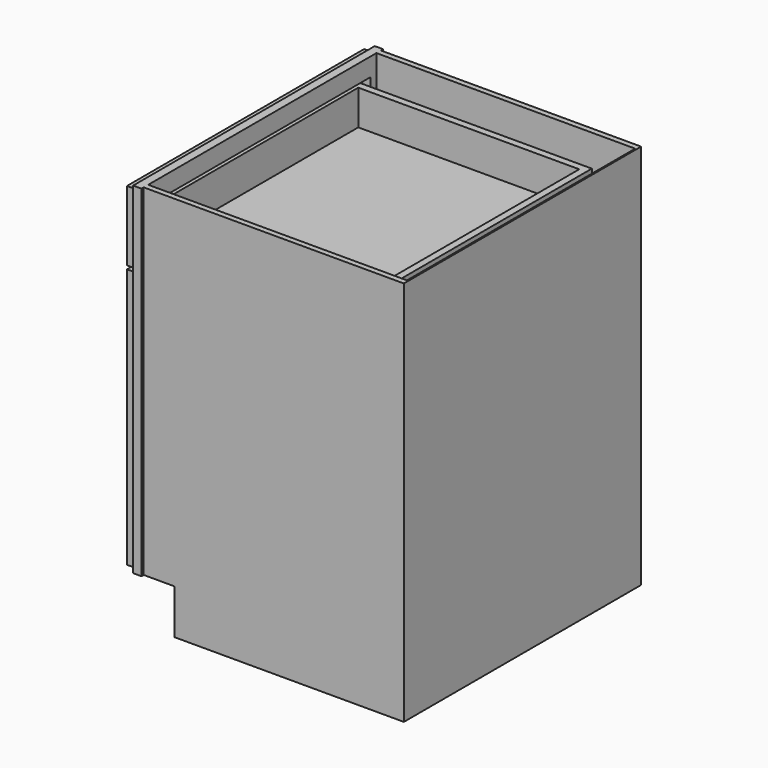
from build123d import *

# Parameters (mm, degrees)
F0_W          = 609.6
F0_H          = 876.3
F1_DEPTH      = 685.8
F2_W          = 88.9
F2_H          = 101.6
F3_DEPTH      = 685.801
F4_W          = 612.7229508197
F4_H          = 692.15
F5_DEPTH      = 19.05
F6_W          = 590.55
F6_H          = 6.35
F7_DEPTH      = 876.301
F8_W          = 587.375
F8_H          = 647.7
F9_DEPTH      = 733.425
F10_W         = 612.7229508197
F10_H         = 41.275
F11_DEPTH     = 19.05
F12_W         = 336.55
F12_H         = 590.5627
F12_W_2       = 222.25
F12_H_2       = 476.2627
F13_DEPTH     = 19.05
F14_W         = 6.35
F14_H         = 222.25
F15_DEPTH     = 476.2627
F16_SIZE      = 3.175
F17_W         = 673.1
F17_H         = 158.75
F17_W_2       = 558.8
F17_H_2       = 82.55
F18_DEPTH     = 19.05
F19_W         = 6.35
F19_H         = 558.8
F20_DEPTH     = 82.55
F21_SIZE      = 3.175
F22_W         = 504.825
F22_H         = 647.7
F23_DEPTH     = 101.6
F24_W         = 584.2
F24_H         = 95.25
F25_DEPTH     = 533.4
F26_T         = 15.875
F26_T3_DEPTH  = 37.249261314
F26_T5_DEPTH  = 37.249261314
F26_T7_DEPTH  = 37.249261314
F26_T9_DEPTH  = 37.249261314
F26_T11_DEPTH = 36.5125
F26_T13_DEPTH = 590.55
F26_T15_DEPTH = 114.3
F26_T17_DEPTH = 127
F26_T19_DEPTH = 615.95
F26_T21_DEPTH = 111.125
F26_T23_DEPTH = 36.5125


# Not quite as in the source:
# - a shell that OpenCascade refuses in one call is made with other operations: the cavity is built on its own and cut out


with BuildPart() as f1:
    # F0 (on Front) → F1 (new body)
    with BuildSketch(Plane.XZ):
        Rectangle(F0_W, F0_H)
    extrude(amount=-F1_DEPTH)

    # F2 (on face) → F3 (cut, through all)
    with BuildSketch(Plane.XZ):
        with Locations((-260.35, -387.35)):
            Rectangle(F2_W, F2_H)
    extrude(amount=-F3_DEPTH, mode=Mode.SUBTRACT)

    # F4 (on face) → F5 (cut)
    with BuildSketch(Plane(origin=(-304.8, 0, 0), x_dir=(0, -1, 0), z_dir=(-1, 0, 0))):
        with Locations((-342.9, 50.8)):
            Rectangle(F4_W, F4_H)
    extrude(amount=-F5_DEPTH, mode=Mode.SUBTRACT)

    # F6 (on face) → F7 (cut, through all)
    with BuildSketch(Plane.XY.offset(438.15)):
        with Locations((9.525, 682.625)):
            Rectangle(F6_W, F6_H)
        with Locations((9.525, 3.175)):
            Rectangle(F6_W, F6_H)
    extrude(amount=-F7_DEPTH, mode=Mode.SUBTRACT)

    # F8 (on face) → F9 (cut, through all)
    with BuildSketch(Plane.XY.offset(438.15)):
        with Locations((7.9375, 342.9)):
            Rectangle(F8_W, F8_H)
    extrude(amount=-F9_DEPTH, mode=Mode.SUBTRACT)

    # F10 (on face) → F11 (join, through all)
    with BuildSketch(Plane(origin=(-304.8, 0, 0), x_dir=(0, -1, 0), z_dir=(-1, 0, 0))):
        with Locations((-342.9, 265.1125)):
            Rectangle(F10_W, F10_H)
    extrude(amount=-F11_DEPTH)

    # F22 (on face) → F23 (cut)
    with BuildSketch(Plane(origin=(0, 0, -438.15), x_dir=(1, 0, 0), z_dir=(0, 0, -1))):
        with Locations((49.2125, -342.9)):
            Rectangle(F22_W, F22_H)
    extrude(amount=-F23_DEPTH, mode=Mode.SUBTRACT)


with BuildPart() as f13:
    # F12 (on face) → F13 (new body)
    with BuildSketch(Plane(origin=(-304.8, 0, 0), x_dir=(0, -1, 0), z_dir=(-1, 0, 0))):
        with Locations((-511.175, -33.33115)):
            Rectangle(F12_W, F12_H)
        with Locations((-511.175, -33.33115)):
            Rectangle(F12_W_2, F12_H_2, mode=Mode.SUBTRACT)
    extrude(amount=F13_DEPTH)

    # F14 (on face) → F15 (join, through all)
    with BuildSketch(Plane.XY.offset(-271.4625)):
        with Locations((-312.7375, 511.175)):
            Rectangle(F14_W, F14_H)
    extrude(amount=F15_DEPTH)

    # F16
    f16_edges = [f13.edges().sort_by_distance(p)[0] for p in [
        (-323.85, 622.3, -33.33115),
        (-323.85, 511.175, -271.4625),
        (-323.85, 400.05, -33.33115),
        (-323.85, 511.175, 204.8002),
    ]]
    chamfer(f16_edges, length=F16_SIZE)


with BuildPart() as f18:
    # F17 (on face) → F18 (new body)
    with BuildSketch(Plane(origin=(-304.8, 0, 0), x_dir=(0, -1, 0), z_dir=(-1, 0, 0))):
        with Locations((-342.9, 349.25)):
            Rectangle(F17_W, F17_H)
        with Locations((-342.9, 349.25)):
            Rectangle(F17_W_2, F17_H_2, mode=Mode.SUBTRACT)
    extrude(amount=F18_DEPTH)

    # F19 (on face) → F20 (join, through all)
    with BuildSketch(Plane.XY.offset(307.975)):
        with Locations((-312.7375, 342.9)):
            Rectangle(F19_W, F19_H)
    extrude(amount=F20_DEPTH)

    # F21
    f21_edges = [f18.edges().sort_by_distance(p)[0] for p in [
        (-323.85, 342.9, 307.975),
        (-323.85, 622.3, 349.25),
        (-323.85, 342.9, 390.525),
        (-323.85, 63.5, 349.25),
    ]]
    chamfer(f21_edges, length=F21_SIZE)

    # F24 (on face) → F25 (join)
    with BuildSketch(Plane.YZ.offset(-304.8)):
        with Locations((342.9, 339.725)):
            Rectangle(F24_W, F24_H)
    extrude(amount=F25_DEPTH)

    # F26: shell of thickness 15.875, made by hand


with BuildPart() as f26_core1:
    # F26_t2: copy of F18
    add(f18.part)

    # the walls: a layer under each face that stays
    f26_faces = [f26_core1.faces().sort_by_distance(p)[0] for p in [
        (-323.85, 567.2666666667, 296.3333333333),
        (-322.2625, 342.9, 306.3875),
        (-322.2625, 61.9125, 349.25),
        (-322.2625, 623.8875, 349.25),
        (-322.2625, 342.9, 392.1125),
        (-314.325, 342.9, 428.625),
        (-314.325, 679.45, 349.25),
        (-314.325, 342.9, 269.875),
        (-314.325, 6.35, 349.25),
        (-318.29375, 342.9, 307.975),
        (-318.29375, 63.5, 349.25),
        (-318.29375, 622.3, 349.25),
        (-318.29375, 342.9, 390.525),
        (-304.8, 567.2666666667, 402.1666666667),
        (-315.9125, 342.9, 349.25),
        (-38.1, 635, 339.725),
        (-38.1, 342.9, 292.1),
        (-38.1, 50.8, 339.725),
        (-307.18125, 63.5, 349.25),
        (-307.18125, 342.9, 390.525),
        (-307.18125, 622.3, 349.25),
        (-304.8, 342.9, 347.6625),
        (228.6, 342.9, 339.725),
        (-307.18125, 342.9, 307.975),
        (-309.5625, 342.9, 349.25),
    ]]
    thicken(f26_faces, amount=-F26_T, mode=Mode.SUBTRACT)

    # F26_s4 → F26_t3 (cut)
    with BuildSketch(Plane(origin=(4.5928978099, 4.5928978099, 4.5928978099), x_dir=(-0.7071067812, 0.7071067812, 0), z_dir=(0.5773502692, 0.5773502692, 0.5773502692))):
        Polygon((271.8908726623, 356.5892701441), (263.7152476623, 342.7036353262), (255.7777476623, 347.2863530879), (255.7777476623, 356.4517886113), align=None)
    extrude(amount=F26_T3_DEPTH, mode=Mode.SUBTRACT)

    # F26_s6 → F26_t5 (cut)
    with BuildSketch(Plane(origin=(-224.0071021901, 224.00710219, -224.0071021901), x_dir=(0.7071067812, 0.7071067812, 0), z_dir=(0.5773502692, -0.5773502692, 0.5773502692))):
        Polygon((213.0429578754, 636.5659477442), (221.2185828754, 622.6803129263), (229.1560828754, 627.263030688), (229.1560828754, 636.4284662114), align=None)
    extrude(amount=F26_T5_DEPTH, mode=Mode.SUBTRACT)

    # F26_s8 → F26_t7 (cut)
    with BuildSketch(Plane(origin=(-228.2404355234, -228.2404355234, 228.2404355234), x_dir=(-0.7071067812, 0.7071067812, 0), z_dir=(0.5773502692, 0.5773502692, -0.5773502692))):
        Polygon((271.8908726623, 213.7335916339), (255.7777476623, 213.8710731668), (255.7777476623, 223.0365086901), (263.7152476623, 227.6192264518), align=None)
    extrude(amount=F26_T7_DEPTH, mode=Mode.SUBTRACT)

    # F26_s10 → F26_t9 (cut)
    with BuildSketch(Plane(origin=(-456.8404355234, 456.8404355234, 456.8404355234), x_dir=(0.7071067812, 0.7071067812, 0), z_dir=(0.5773502692, -0.5773502692, -0.5773502692))):
        Polygon((213.0429578754, -66.2430859662), (229.1560828754, -66.1056044334), (229.1560828754, -56.94016891), (221.2185828754, -52.3574511483), align=None)
    extrude(amount=F26_T9_DEPTH, mode=Mode.SUBTRACT)

    # F26_s12 → F26_t11 (cut)
    with BuildSketch(Plane.YZ.offset(-336.55)):
        Polygon((622.14125, 308.13375), (622.3, 292.1), (638.175, 292.1), (638.175, 307.975), align=None)
        Polygon((63.65875, 308.13375), (63.5, 292.1), (47.625, 292.1), (47.625, 307.975), align=None)
        Polygon((63.65875, 390.36625), (47.625, 390.525), (47.625, 406.4), (63.5, 406.4), align=None)
        Polygon((622.14125, 390.36625), (638.175, 390.525), (638.175, 406.4), (622.3, 406.4), align=None)
    extrude(amount=F26_T11_DEPTH, mode=Mode.SUBTRACT)

    # F26_s14 → F26_t13 (cut)
    with BuildSketch(Plane.XZ.offset(-638.175)):
        Polygon((-316.07125, 308.13375), (-315.9125, 292.1), (-300.0375, 292.1), (-300.0375, 307.975), align=None)
        Polygon((-316.07125, 390.36625), (-315.9125, 406.4), (-300.0375, 406.4), (-300.0375, 390.525), align=None)
        Polygon((-309.40375, 390.36625), (-309.5625, 406.4), (-325.4375, 406.4), (-325.4375, 390.525), align=None)
        Polygon((-304.95875, 308.13375), (-288.925, 307.975), (-288.925, 292.1), (-304.8, 292.1), align=None)
        Polygon((-309.40375, 308.13375), (-309.5625, 292.1), (-325.4375, 292.1), (-325.4375, 307.975), align=None)
    extrude(amount=F26_T13_DEPTH, mode=Mode.SUBTRACT)

    # F26_s16 → F26_t15 (cut)
    with BuildSketch(Plane.XY.offset(292.1)):
        Polygon((-316.07125, 63.65875), (-315.9125, 47.625), (-300.0375, 47.625), (-300.0375, 63.5), align=None)
        Polygon((-316.07125, 622.14125), (-315.9125, 638.175), (-300.0375, 638.175), (-300.0375, 622.3), align=None)
        Polygon((-309.40375, 63.65875), (-309.5625, 47.625), (-325.4375, 47.625), (-325.4375, 63.5), align=None)
        Polygon((-309.40375, 622.14125), (-309.5625, 638.175), (-325.4375, 638.175), (-325.4375, 622.3), align=None)
    extrude(amount=F26_T15_DEPTH, mode=Mode.SUBTRACT)

    # F26_s18 → F26_t17 (cut)
    with BuildSketch(Plane.XY.offset(276.225)):
        Polygon((-304.64125, 635.15875), (-320.675, 635), (-320.675, 619.125), (-304.8, 619.125), align=None)
        Polygon((-304.64125, 50.64125), (-320.675, 50.8), (-320.675, 66.675), (-304.8, 66.675), align=None)
    extrude(amount=F26_T17_DEPTH, mode=Mode.SUBTRACT)

    # F26_s20 → F26_t19 (cut)
    with BuildSketch(Plane.XZ.offset(-650.875)):
        Polygon((-304.64125, 291.94125), (-320.675, 292.1), (-320.675, 307.975), (-304.8, 307.975), align=None)
    extrude(amount=F26_T19_DEPTH, mode=Mode.SUBTRACT)

    # F26_s22 → F26_t21 (cut)
    with BuildSketch(Plane.XY.offset(292.1)):
        Polygon((-304.95875, 63.65875), (-304.8, 47.625), (-288.925, 47.625), (-288.925, 63.5), align=None)
        Polygon((-304.95875, 622.14125), (-304.8, 638.175), (-288.925, 638.175), (-288.925, 622.3), align=None)
    extrude(amount=F26_T21_DEPTH, mode=Mode.SUBTRACT)

    # F26_s24 → F26_t23 (cut)
    with BuildSketch(Plane.YZ.offset(-325.4375)):
        Polygon((63.65875, 308.13375), (47.625, 307.975), (47.625, 292.1), (63.5, 292.1), align=None)
        Polygon((63.65875, 390.36625), (47.625, 390.525), (47.625, 406.4), (63.5, 406.4), align=None)
        Polygon((622.14125, 390.36625), (622.3, 406.4), (638.175, 406.4), (638.175, 390.525), align=None)
        Polygon((622.14125, 308.13375), (638.175, 307.975), (638.175, 292.1), (622.3, 292.1), align=None)
    extrude(amount=F26_T23_DEPTH, mode=Mode.SUBTRACT)


with BuildPart() as f18_1:
    add(f18.part)

    # what is left inside the walls is the cavity
    f26_cavity = [f26_core1.part.solids().sort_by_distance(p)[0] for p in [
        (45.508333, 342.9, 308.13375),
    ]]
    add(f26_cavity, mode=Mode.SUBTRACT)


with BuildPart() as f27_1:
    # F27: instance of F13
    add(f13.part.mirror(Plane(origin=(-314.325, 342.9, -33.33115), x_dir=(1, 0, 0), z_dir=(0, -1, 0))))


solid = Compound([f1.part, f13.part, f18_1.part, f27_1.part])
